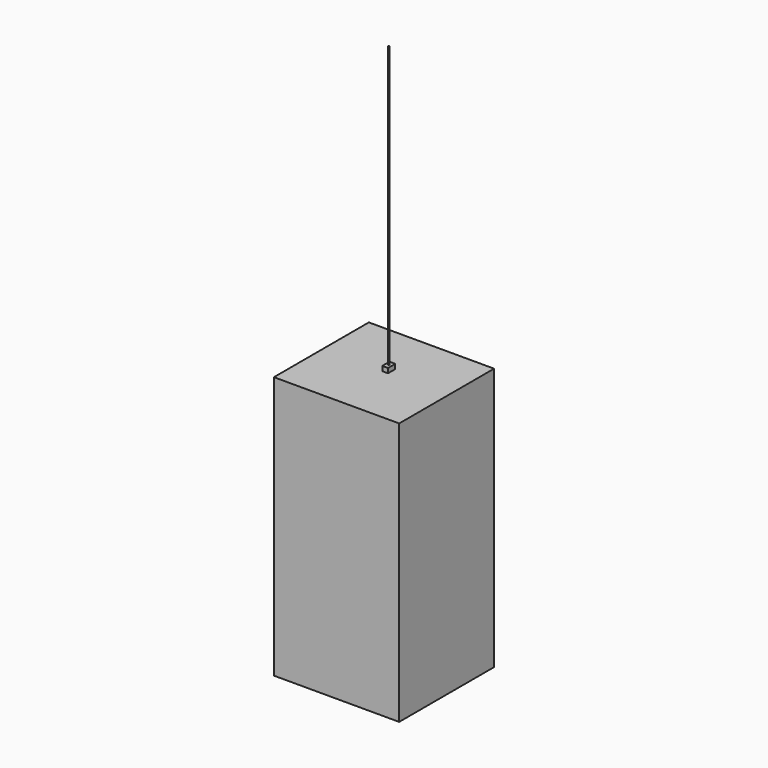
from build123d import *

# Parameters (mm, degrees)
F0_W     = 26.815738529
F0_H     = 56.2547557056
F1_DEPTH = 25.4
F2_W     = 18.9459016547
F2_H     = 11.3675417379
F3_DEPTH = 12.5
F4_W     = 1.2322755065
F4_H     = 1.9270461053
F5_DEPTH = 1
F6_R     = 0.1393490387
F7_DEPTH = 60


# Not quite as in the source:
# - a feature names something its author has since deleted; it is built from what else it names


with BuildPart() as f1:
    # F0 (on Front) → F1 (new body)
    with BuildSketch(Plane.XZ):
        Rectangle(F0_W, F0_H)
    extrude(amount=F1_DEPTH)

    # F2 (on face) → F3 (cut, symmetric)
    with BuildSketch(Plane(origin=(0, 0, -28.1273778528), x_dir=(1, 0, 0), z_dir=(0, 0, -1))):
        with Locations((0.7286877371, 11.9504923932)):
            Rectangle(F2_W, F2_H)
    extrude(amount=F3_DEPTH, both=True, mode=Mode.SUBTRACT)

    # F4 (on face) → F5 (join)
    with BuildSketch(Plane.XY.offset(28.1273778528)):
        with Locations((0, -11.4252325147)):
            Rectangle(F4_W, F4_H)
    extrude(amount=F5_DEPTH)

    # F6 (on face) → F7 (join)
    with BuildSketch(Plane.XY.offset(29.1273778528)):
        with Locations((0, -11.4126661792)):
            Circle(F6_R)
    extrude(amount=F7_DEPTH)


solid = f1.part
